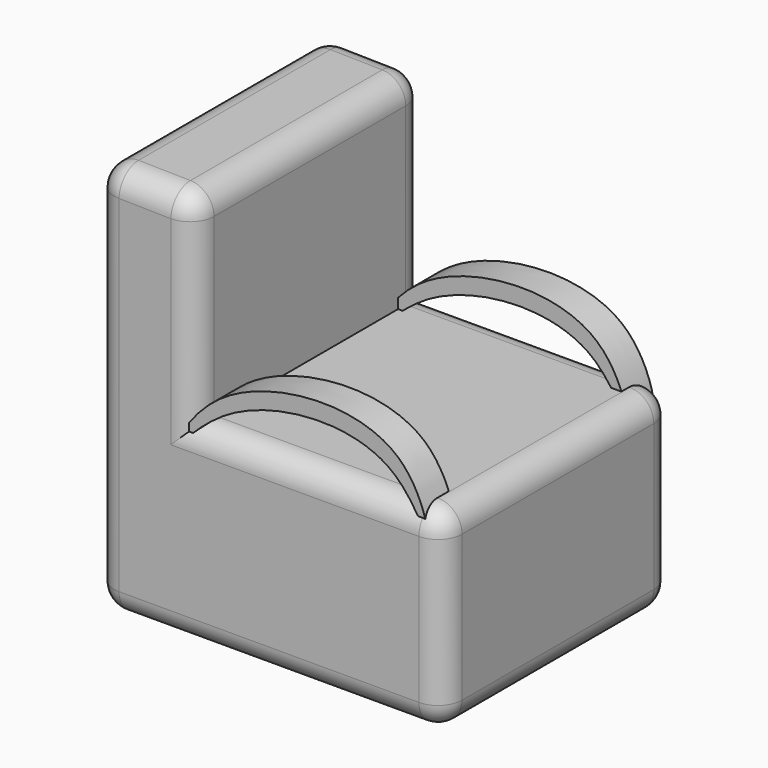
from build123d import *

# Parameters (mm, degrees)
F1_DEPTH = 60
F2_R     = 5
F4_DEPTH = 7


with BuildPart() as f1:
    # F0 (on Front) → F1 (new body)
    with BuildSketch(Plane.XZ):
        Polygon((-16.3266230375, 46.3065057993), (-37.1406786144, 46.6884113848), (-37.1406786144, -35.6130450964), (35.4220867157, -35.6130450964), (35.4220867157, 4.8693437129), (-16.3266230375, 4.8693437129), align=None)
    extrude(amount=F1_DEPTH)

    # F2
    f2_edges = [f1.edges().sort_by_distance(p)[0] for p in [
        (-26.733651, -60, 46.497459),
        (-16.326623, -60, 25.587925),
        (-37.140679, -60, 5.537683),
        (-0.859296, -60, -35.613045),
        (35.422087, -60, -15.371851),
        (9.547732, -60, 4.869344),
        (-37.140679, -30, 46.688411),
        (-37.140679, 0, 5.537683),
        (-16.326623, 0, 25.587925),
        (9.547732, 0, 4.869344),
        (35.422087, 0, -15.371851),
        (-0.859296, 0, -35.613045),
        (35.422087, -30, -35.613045),
        (35.422087, -30, 4.869344),
        (-16.326623, -30, 46.306506),
        (-37.140679, -30, -35.613045),
        (-26.733651, 0, 46.497459),
    ]]
    fillet(f2_edges, radius=F2_R)



with BuildPart() as f4:
    # F3 (on Front) → F4 (new body)
    with BuildSketch(Plane.XZ):
        with BuildLine():
            add(Edge.make_bspline(
                [(-20.5802507699, 0), (-21.0227503672, 0.3645522021), (-12.8309139993, 17.1634287), (27.8504452332, 20.6433461702), (33.2120306515, -6.999396719), (24.8552818153, 16.4532725506), (-10.2450219104, 13.6545194096), (-20.1484695003, -0.3557219341), (-20.5802507699, 0)],
                knots=[0, 0, 0, 0, 0.1425055416, 0.3701759996, 0.5106067058, 0.6428437051, 0.8609462606, 1, 1, 1, 1], degree=3))
        make_face()
    extrude(amount=F4_DEPTH)


with BuildPart() as f1_1:
    add(f1.part)

    add(f4.part)  # F6 merges F4
    # F6: F4 across plane
    add(f4.part.mirror(Plane.XZ.offset(29.5)))


solid = f1_1.part
